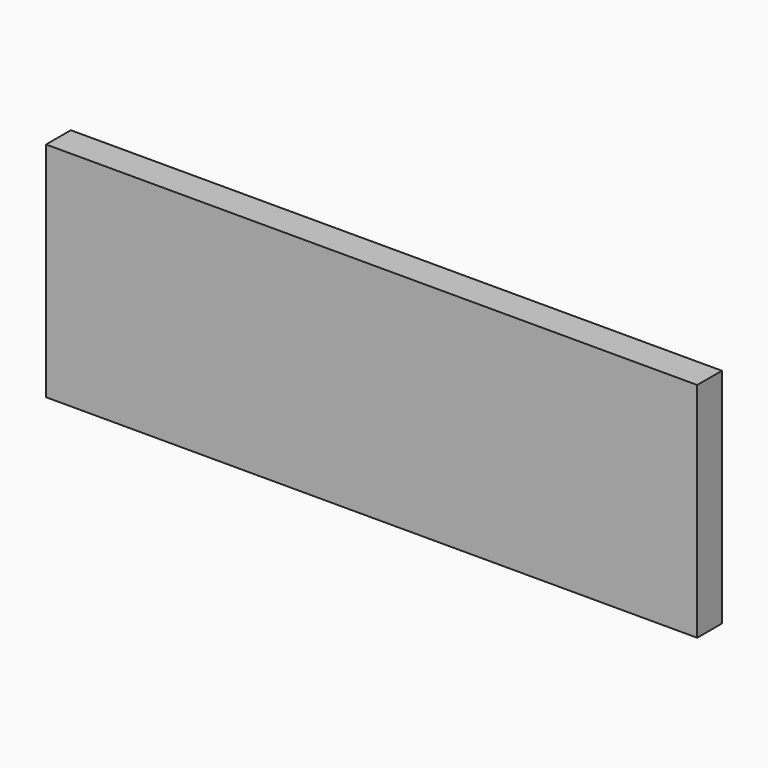
from build123d import *

# Parameters (mm, degrees)
F0_W     = 59.0336769819
F0_H     = 20.1775263995
F1_DEPTH = 2.8


# Not quite as in the source:
# - the program builds the solid bodies; features that only make, move or delete a surface that nothing else refers to are left out


with BuildPart() as f1:
    # F0 (on Front) → F1 (new body)
    with BuildSketch(Plane.XZ):
        with Locations((-29.516838491, -10.0887631997)):
            Rectangle(F0_W, F0_H)
    extrude(amount=F1_DEPTH)


solid = f1.part
